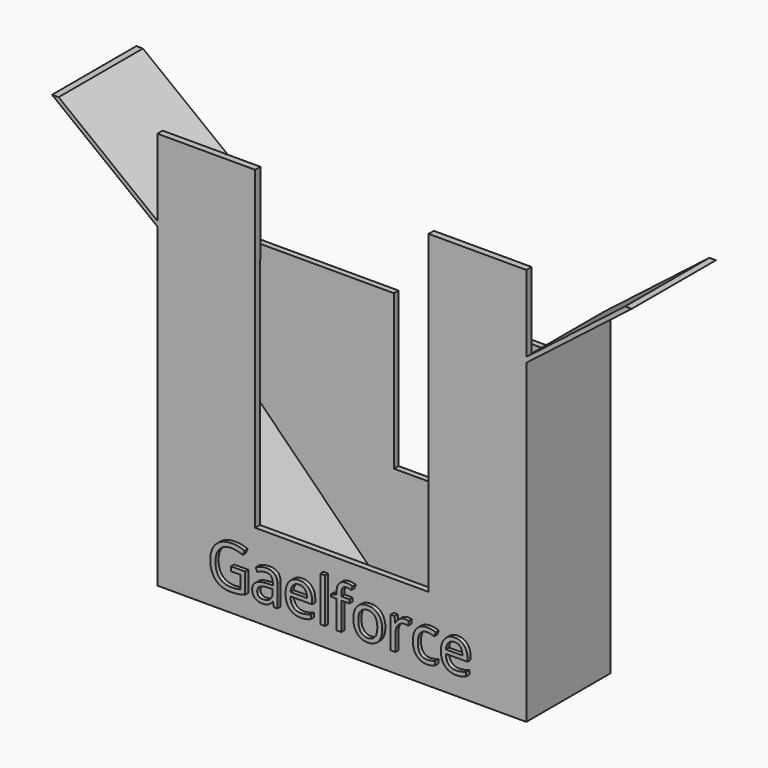
from build123d import *

# Parameters (mm, degrees)
F0_W         = 355.6
F0_H         = 304.8
F1_DEPTH     = 50.8
F2_W         = 342.9
F2_H         = 90.17
F3_DEPTH     = 292.1
F4_W         = 342.9
F4_H         = 5.5685455938
F5_DEPTH     = 46.482
F6_W         = 167.1909952334
F6_H         = 225.065162268
F7_DEPTH     = 25.4
F8_TEXT_SIZE = 56.7017019623
F9_DEPTH     = 3.81
F10_W        = 53.218498826
F10_H        = 148.9302129619
F11_DEPTH    = 25.4
F12_SIZE     = 127
F14_DEPTH    = 101.6
F16_DEPTH    = 159.258
F15_W        = 167.1909952334
F15_H        = 78.770831532
F17_DEPTH    = 313.182
F19_DEPTH    = 95.25


# Not quite as in the source:
# - Text() gives the source's letters only with a copy of the font that has no kerning and outlines rounded to 1/6400 em; it was checked with that copy


with BuildPart() as f1:
    # F0 (on Front) → F1 (new body, symmetric)
    with BuildSketch(Plane.XZ):
        Rectangle(F0_W, F0_H)
    extrude(amount=F1_DEPTH, both=True)

    # F2 (on face) → F3 (cut)
    with BuildSketch(Plane.XY.offset(152.4)):
        with Locations((0, 0.1464544062)):
            Rectangle(F2_W, F2_H)
    extrude(amount=-F3_DEPTH, mode=Mode.SUBTRACT)

    # F4 (on face) → F5 (cut)
    with BuildSketch(Plane.XY.offset(152.4)):
        with Locations((0, 48.0157272031)):
            Rectangle(F4_W, F4_H)
    extrude(amount=-F5_DEPTH, mode=Mode.SUBTRACT)

    # F6 (on face) → F7 (cut)
    with BuildSketch(Plane.XZ.offset(50.8)):
        with Locations((0, 264.932581134)):
            Rectangle(F6_W, F6_H)
        with Locations((0, 39.867418866)):
            Rectangle(F6_W, F6_H)
    extrude(amount=-F7_DEPTH, mode=Mode.SUBTRACT)

    # F10 (on face) → F11 (cut)
    with BuildSketch(Plane(origin=(0, 50.8, 0), x_dir=(-1, 0, 0), z_dir=(0, 1, 0))):
        with Locations((0, 31.452893519)):
            Rectangle(F10_W, F10_H)
    extrude(amount=-F11_DEPTH, mode=Mode.SUBTRACT)

    # F12
    f12_edges = [f1.edges().sort_by_distance(p)[0] for p in [
        (-171.45, 0.146454, -139.7),
        (171.45, 0.146454, -139.7),
    ]]
    chamfer(f12_edges, length=F12_SIZE)

    # F13 (on face) → F14 (join)
    with BuildSketch(Plane.XZ.offset(50.8)):
        Polygon((-279.4, 231.170831532), (-279.4, 152.4), (-177.8, 152.4), (-83.5954976167, 152.4), (83.5954976167, 152.4), (177.8, 152.4), (279.4, 152.4), (279.4, 231.170831532), align=None)
    extrude(amount=-F14_DEPTH)

    # F15 (on face) → F16 (cut)
    with BuildSketch(Plane.XZ.offset(50.8)):
        Polygon((-279.4, 152.4), (-177.8, 152.4), (-279.4, 231.170831532), align=None)
        Polygon((279.4, 231.170831532), (177.8, 152.4), (279.4, 152.4), align=None)
        Polygon((177.8, 231.170831532), (177.8, 157.3231769708), (273.05, 231.170831532), align=None)
        Polygon((-273.05, 231.170831532), (-177.8, 157.3231769708), (-177.8, 231.170831532), align=None)
    extrude(amount=-F16_DEPTH, mode=Mode.SUBTRACT)

    # F15 (on face) → F17 (cut)
    with BuildSketch(Plane.XZ.offset(50.8)):
        with Locations((0, 191.785415766)):
            Rectangle(F15_W, F15_H)
    extrude(amount=-F17_DEPTH, mode=Mode.SUBTRACT)

    # F18 (on face) → F19 (cut)
    with BuildSketch(Plane(origin=(0, 50.8, 0), x_dir=(-1, 0, 0), z_dir=(0, 1, 0))):
        Polygon((-177.8, 231.170831532), (-177.8, 157.3231769708), (-171.45, 152.4), (-83.5954976167, 152.4), (-83.5954976167, 231.170831532), align=None)
        Polygon((83.5954976167, 231.170831532), (83.5954976167, 152.4), (171.45, 152.4), (177.8, 157.3231769708), (177.8, 231.170831532), align=None)
    extrude(amount=-F19_DEPTH, mode=Mode.SUBTRACT)


with BuildPart() as f9:
    # F8 (on face) → F9 (new body)
    with BuildSketch(Plane.XZ.offset(50.8)):
        with Locations((-127.2470392287, -131.6035613418)):
            Text('Gaelforce', F8_TEXT_SIZE, font='Open Sans', text_align=(TextAlign.LEFT, TextAlign.BOTTOM))
    extrude(amount=F9_DEPTH)


solid = Compound([f1.part, f9.part])
